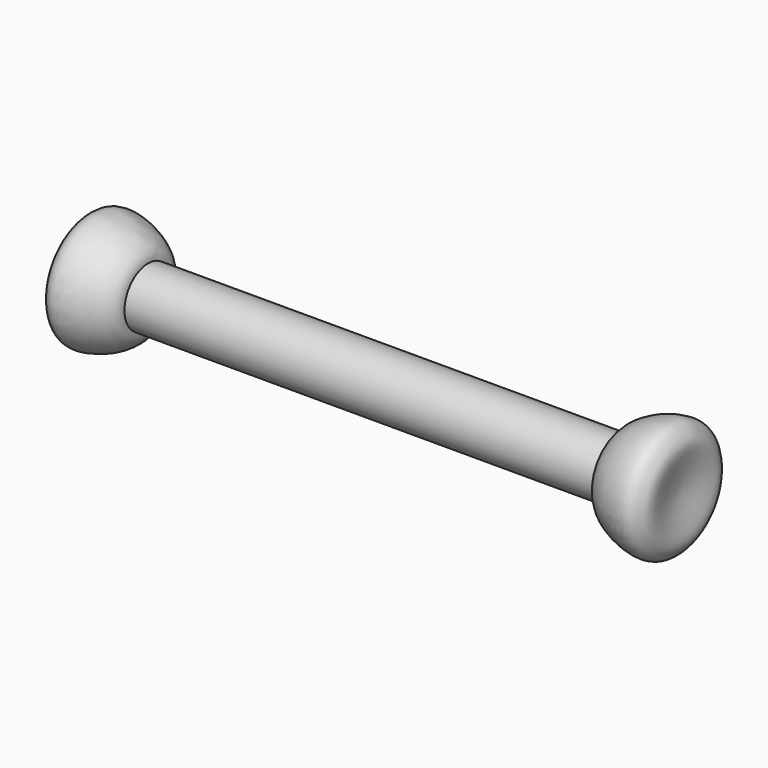
from build123d import *

# Parameters (mm, degrees)
F1_R     = 25
F2_DEPTH = 200


# Not quite as in the source:
# - a pattern or mirror of a feature is missing from the dataset's text; its kind, count and spacing are read off the source's solid


with BuildPart() as f2:
    # F1 (on Right) → F2 (new body, symmetric)
    with BuildSketch(Plane.YZ):
        Circle(F1_R)
    extrude(amount=F2_DEPTH, both=True)

    # F3 (on Front) → F4 (revolve)
    with BuildSketch(Plane.XZ):
        with BuildLine():
            add(Edge.make_bspline(
                [(200, 25), (199.201641866, 39.0983767897), (241.4136147213, 55.7899440033), (251.4561134334, 44.2516899933), (257.9215918294, 33.9973185388), (250, 13.5196693598), (250, 0)],
                knots=[0, 0, 0, 0, 0.3500294963, 0.535933113, 0.6975420206, 1, 1, 1, 1], degree=3))
            Line((200, 25), (200, 0))
            Line((200, 0), (250, 0))
        make_face()
    f4 = revolve(axis=Axis((225, 0, 0), (1, 0, 0)))

    # F4_copies: F4 across plane
    add(f4.mirror(Plane(origin=(0, 0, 0), x_dir=(0, 0, -1), z_dir=(-1, 0, 0))))


solid = f2.part
